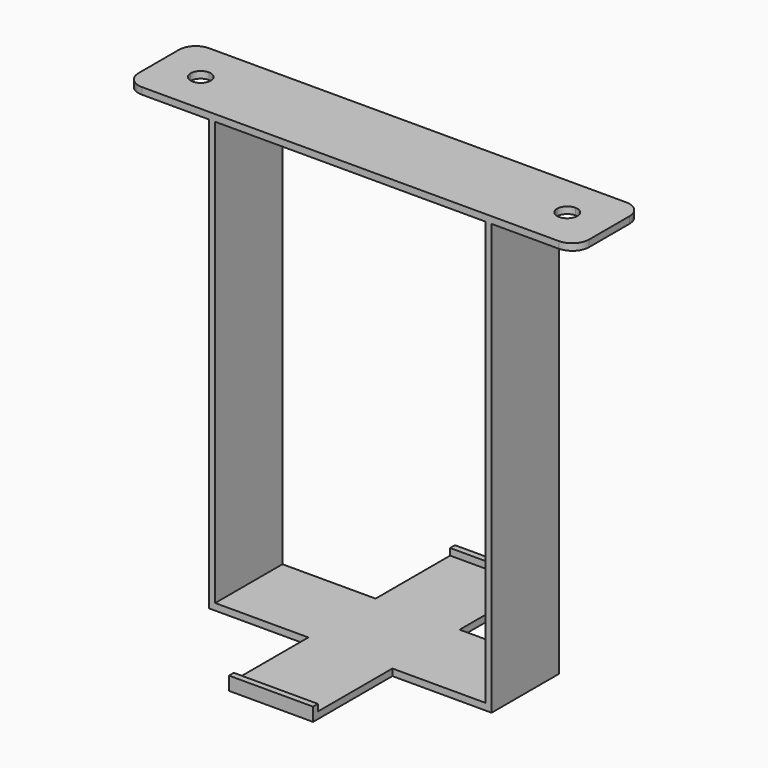
from build123d import *

# Parameters (mm, degrees)
F0_W      = 25
F0_H      = 27.7
F0_H_2    = 25
F0_W_2    = 27.7
F1_DEPTH  = 2
F0_W_3    = 1.8
F2_DEPTH  = 130
F0_H_3    = 1.8
F3_DEPTH  = 4
F4_W      = 25
F4_H      = 2
F5_DEPTH  = 80.4
F7_W      = 25
F7_H      = 2
F8_DEPTH  = 25
F6_W      = 25
F6_H      = 2
F9_DEPTH  = 25
F12_DEPTH = 25
F13_R     = 5


with BuildPart() as f1:
    # F0 (on Top) → F1 (new body)
    with BuildSketch(Plane.XY):
        with Locations((0, 26.35)):
            Rectangle(F0_W, F0_H)
        Rectangle(F0_W, F0_H_2)
        with Locations((26.35, 0)):
            Rectangle(F0_W_2, F0_H_2)
        with Locations((0, -26.35)):
            Rectangle(F0_W, F0_H)
        with Locations((-26.35, 0)):
            Rectangle(F0_W_2, F0_H_2)
    extrude(amount=F1_DEPTH)

    # F0 (on Top) → F2 (join)
    with BuildSketch(Plane.XY):
        with Locations((-41.1, 0)):
            Rectangle(F0_W_3, F0_H_2)
        with Locations((41.1, 0)):
            Rectangle(F0_W_3, F0_H_2)
    extrude(amount=F2_DEPTH)

    # F0 (on Top) → F3 (join)
    with BuildSketch(Plane.XY):
        with Locations((0, 41.1)):
            Rectangle(F0_W, F0_H_3)
        with Locations((0, -41.1)):
            Rectangle(F0_W, F0_H_3)
    extrude(amount=F3_DEPTH)

    # F4 (on face) → F5 (join)
    with BuildSketch(Plane(origin=(40.2, 0, 0), x_dir=(0, -1, 0), z_dir=(-1, 0, 0))):
        with Locations((0, 129)):
            Rectangle(F4_W, F4_H)
    extrude(amount=F5_DEPTH)

    # F7 (on face) → F8 (join)
    with BuildSketch(Plane.YZ.offset(42)):
        with Locations((0, 129)):
            Rectangle(F7_W, F7_H)
    extrude(amount=F8_DEPTH)

    # F6 (on face) → F9 (join)
    with BuildSketch(Plane(origin=(-42, 0, 0), x_dir=(0, -1, 0), z_dir=(-1, 0, 0))):
        with Locations((0, 129)):
            Rectangle(F6_W, F6_H)
    extrude(amount=F9_DEPTH)

    # F11 (on face) + F10 (on face) → F12 (cut)
    with BuildSketch(Plane(origin=(0, 0, 128), x_dir=(1, 0, 0), z_dir=(0, 0, -1))):
        with BuildLine():
            ThreePointArc((-51.5, 0), (-52.3786796564, 2.1213203436), (-54.5, 3))
            Line((-54.5, 3), (-54.5, 0))
            Line((-54.5, 0), (-51.5, 0))
        make_face()
        with BuildLine():
            Line((-54.5, 0), (-54.5, 3))
            ThreePointArc((-54.5, 3), (-56.6213203436, 2.1213203436), (-57.5, 0))
            Line((-57.5, 0), (-54.5, 0))
        make_face()
        with BuildLine():
            Line((-51.5, 0), (-54.5, 0))
            Line((-54.5, 0), (-54.5, -3))
            ThreePointArc((-54.5, -3), (-52.3786796564, -2.1213203436), (-51.5, 0))
        make_face()
        with BuildLine():
            Line((-54.5, -3), (-54.5, 0))
            Line((-54.5, 0), (-57.5, 0))
            ThreePointArc((-57.5, 0), (-56.6213203436, -2.1213203436), (-54.5, -3))
        make_face()
    with BuildSketch(Plane(origin=(0, 0, 128), x_dir=(1, 0, 0), z_dir=(0, 0, -1))):
        with BuildLine():
            Line((54.5, 0), (54.5, 3))
            ThreePointArc((54.5, 3), (52.3786796564, 2.1213203436), (51.5, 0))
            Line((51.5, 0), (54.5, 0))
        make_face()
        with BuildLine():
            ThreePointArc((57.5, 0), (56.6213203436, 2.1213203436), (54.5, 3))
            Line((54.5, 3), (54.5, 0))
            Line((54.5, 0), (57.5, 0))
        make_face()
        with BuildLine():
            Line((57.5, 0), (54.5, 0))
            Line((54.5, 0), (54.5, -3))
            ThreePointArc((54.5, -3), (56.6213203436, -2.1213203436), (57.5, 0))
        make_face()
        with BuildLine():
            Line((54.5, -3), (54.5, 0))
            Line((54.5, 0), (51.5, 0))
            ThreePointArc((51.5, 0), (52.3786796564, -2.1213203436), (54.5, -3))
        make_face()
    extrude(amount=-F12_DEPTH, mode=Mode.SUBTRACT)

    # F13
    f13_edges = [f1.edges().sort_by_distance(p)[0] for p in [
        (67, 12.5, 129),
        (67, -12.5, 129),
        (-67, 12.5, 129),
        (-67, -12.5, 129),
    ]]
    fillet(f13_edges, radius=F13_R)


solid = f1.part
